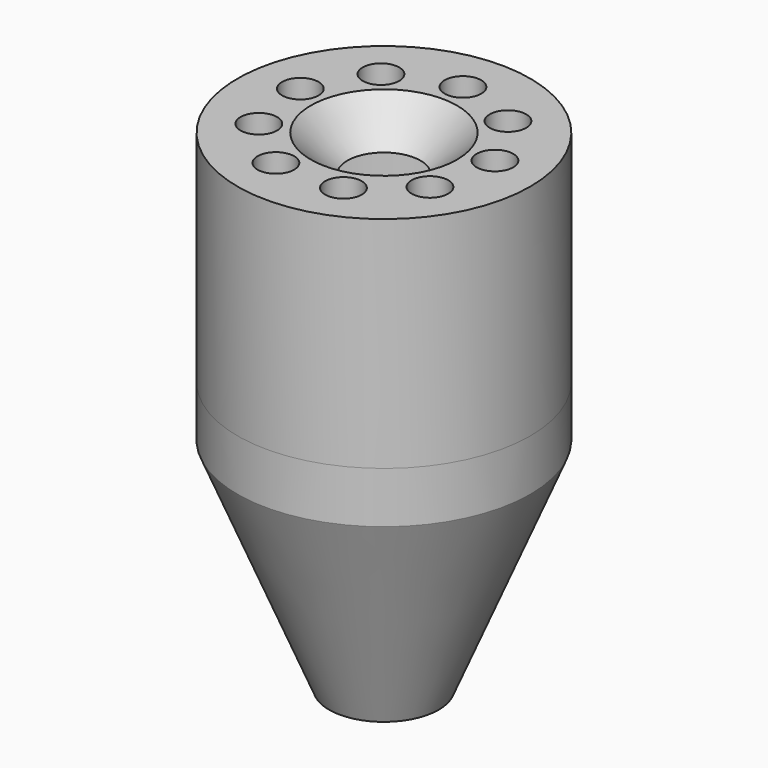
from build123d import *

# Parameters (mm, degrees)
F1_R      = 25.4
F2_R      = 9.525
F4_R      = 22.225
F5_R      = 6.35
F7_DEPTH  = 8.89
F8_R      = 6.35
F9_DEPTH  = 8.89
F8_R_2    = 25.4
F10_DEPTH = 38.1
F13_SIZE  = 6.34999
F14_R     = 3.175
F15_DEPTH = 38.1


# Not quite as in the source:
# - a fillet or chamfer is up to 0.001 mm smaller than in the source, because OpenCascade refuses the exact size


with BuildPart() as f3:
    # F1 (on offset) → F3 section 0
    with BuildSketch(Plane.XY.offset(38.1)):
        Circle(F1_R)
    # F2 (on Top) → F3 section 1
    with BuildSketch(Plane.XY):
        Circle(F2_R)
    loft()

    # F4 (on face) → F6 section 0
    with BuildSketch(Plane.XY.offset(38.1)):
        Circle(F4_R)
    # F5 (on face) → F6 section 1
    with BuildSketch(Plane.XY):
        Circle(F5_R)
    loft(mode=Mode.SUBTRACT)

    # F1 (on offset) → F7 (join)
    with BuildSketch(Plane.XY.offset(38.1)):
        Circle(F1_R)
    extrude(amount=F7_DEPTH)

    # F8 (on face) → F9 (cut, through all)
    with BuildSketch(Plane.XY.offset(46.99)):
        Circle(F8_R)
    extrude(amount=-F9_DEPTH, mode=Mode.SUBTRACT)


with BuildPart() as f10:
    # F8 (on face) → F10 (new body)
    with BuildSketch(Plane.XY.offset(46.99)):
        Circle(F8_R_2)
        Circle(F8_R, mode=Mode.SUBTRACT)
    extrude(amount=F10_DEPTH)

    # F11 (on Front) → F12 (revolve, cut)
    with BuildSketch(Plane.XZ):
        with BuildLine():
            ThreePointArc((20.32, 75.565), (19.3900640303, 77.8100640303), (17.145, 78.74))
            Line((17.145, 78.74), (0, 78.74))
            Line((0, 78.74), (0, 53.34))
            Line((0, 53.34), (17.145, 53.34))
            ThreePointArc((17.145, 53.34), (19.3900640303, 54.2699359697), (20.32, 56.515))
            Line((20.32, 56.515), (20.32, 75.565))
        make_face()
    revolve(axis=Axis((0, 0, 85.09), (0, 0, 1)), mode=Mode.SUBTRACT)

    # F13 (size 6.35 in the source; OpenCascade refuses exactly that, so slightly less here)
    f13_edges = [f10.edges().sort_by_distance(p)[0] for p in [
        (-6.35, 0, 46.99),
        (-6.35, 0, 85.09),
    ]]
    chamfer(f13_edges, length=F13_SIZE)

    # F14 (on face) → F15 (cut, through all)
    with BuildSketch(Plane.XY.offset(85.09)):
        with Locations((0, 17.145)):
            Circle(F14_R)
        with Locations((-11.0205935681, 13.1338319773)):
            Circle(F14_R)
        with Locations((-16.8845289254, 2.9771980061)):
            Circle(F14_R)
        with Locations((-14.8480055479, -8.5725)):
            Circle(F14_R)
        with Locations((-5.8639353573, -16.1110299834)):
            Circle(F14_R)
        with Locations((5.8639353573, -16.1110299834)):
            Circle(F14_R)
        with Locations((14.8480055479, -8.5725)):
            Circle(F14_R)
        with Locations((16.8845289254, 2.9771980061)):
            Circle(F14_R)
        with Locations((11.0205935681, 13.1338319773)):
            Circle(F14_R)
    extrude(amount=-F15_DEPTH, mode=Mode.SUBTRACT)


solid = Compound([f3.part, f10.part])
